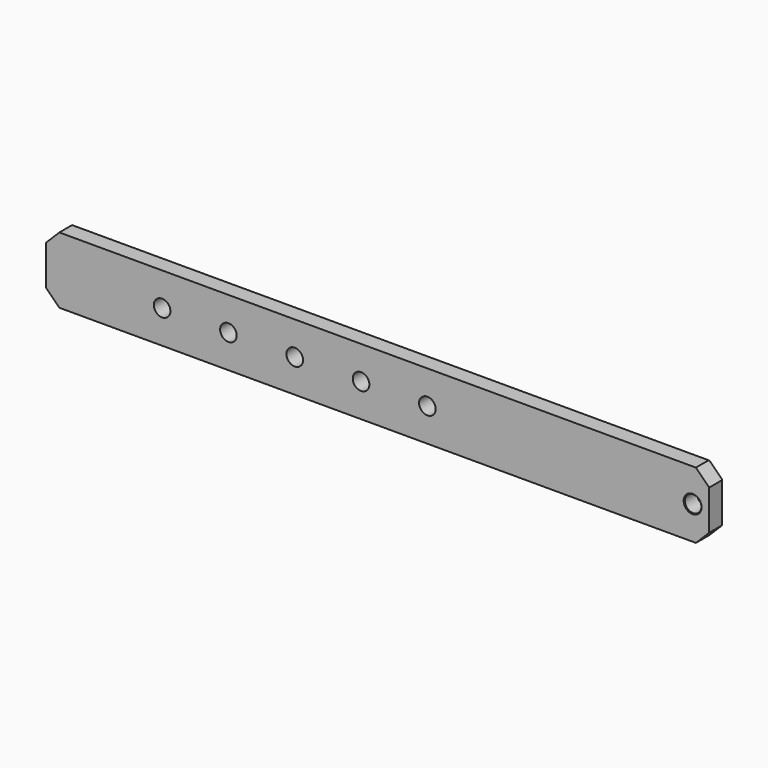
from build123d import *

# Parameters (mm, degrees)
F0_W        = 254
F0_H        = 25.4
F0_R        = 3.175
F1_DEPTH    = 6.35
F2_SIZE     = 0.254
F3_T1_DEPTH = 32.2242991577


# Not quite as in the source:
# - a fillet or chamfer that OpenCascade refuses, or shapes differently, is made with other operations: its cross-section is extruded or revolved along the edge and cut away or added
# - a feature names something its author has since deleted; it is built from what else it names


with BuildPart() as f1:
    # F0 (on Front) → F1 (new body)
    with BuildSketch(Plane.XZ):
        Rectangle(F0_W, F0_H)
        with Locations((-82.55, 0)):
            Circle(F0_R, mode=Mode.SUBTRACT)
        with Locations((-57.15, 0)):
            Circle(F0_R, mode=Mode.SUBTRACT)
        with Locations((-31.75, 0)):
            Circle(F0_R, mode=Mode.SUBTRACT)
        with Locations((-6.35, 0)):
            Circle(F0_R, mode=Mode.SUBTRACT)
        with Locations((19.05, 0)):
            Circle(F0_R, mode=Mode.SUBTRACT)
        with Locations((120.65, 0)):
            Circle(F0_R, mode=Mode.SUBTRACT)
    extrude(amount=F1_DEPTH)

    # F2
    f2_edges = [f1.edges().sort_by_distance(p)[0] for p in [
        (117.475, -6.35, 0),
        (117.475, 0, 0),
        (0, 0, -12.7),
        (127, 0, 0),
        (0, 0, 12.7),
        (-127, 0, 0),
        (-85.725, 0, 0),
        (-60.325, 0, 0),
        (-34.925, 0, 0),
        (-9.525, 0, 0),
        (15.875, 0, 0),
    ]]
    chamfer(f2_edges, length=F2_SIZE)

    # F3: chamfer of 5.08 on 4 edges, made by hand

    # F3_s2 → F3_t1 (cut)
    with BuildSketch(Plane.XZ.offset(-12.8101495789)):
        Polygon((-127, 7.62), (-121.92, 12.7), (-127, 12.7), align=None)
        Polygon((127, 7.62), (121.92, 12.7), (127, 12.7), align=None)
        Polygon((121.92, -12.7), (127, -7.62), (127, -12.7), align=None)
        Polygon((-121.92, -12.7), (-127, -7.62), (-127, -12.7), align=None)
    extrude(amount=F3_T1_DEPTH, mode=Mode.SUBTRACT)


solid = f1.part
